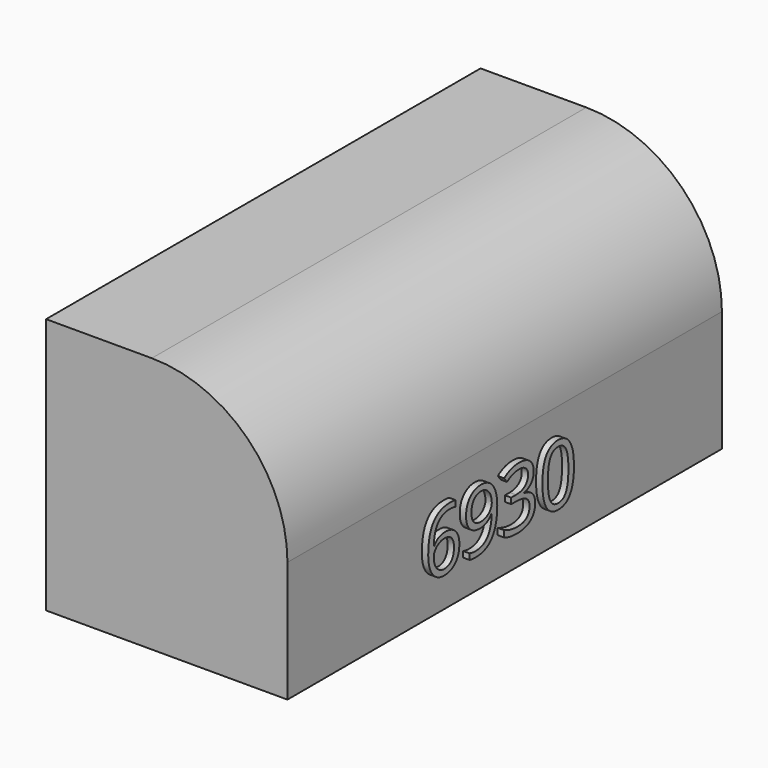
from build123d import *

# Parameters (mm, degrees)
F0_W         = 80
F0_H         = 85
F1_DEPTH     = 180
F2_R         = 44.9488662161
F3_TEXT_SIZE = 27.7048908174
F4_DEPTH     = 2.1


# Not quite as in the source:
# - Text() gives the source's letters only with a copy of the font that has no kerning and outlines rounded to 1/6400 em; it was checked with that copy


with BuildPart() as f1:
    # F0 (on Front) → F1 (new body)
    with BuildSketch(Plane.XZ):
        with Locations((-14.8788882699, -30.3088780493)):
            Rectangle(F0_W, F0_H)
    extrude(amount=F1_DEPTH)

    # F2
    f2_edges = [f1.edges().sort_by_distance(p)[0] for p in [
        (25.121112, -90, 12.191122),
    ]]
    fillet(f2_edges, radius=F2_R)

    # F3 (on face) → F4 (join)
    with BuildSketch(Plane.YZ.offset(25.1211117301)):
        with Locations((-125.8957982063, -60.9868690372)):
            Text('6930', F3_TEXT_SIZE, font='Open Sans', text_align=(TextAlign.LEFT, TextAlign.BOTTOM))
    extrude(amount=F4_DEPTH)


solid = f1.part
